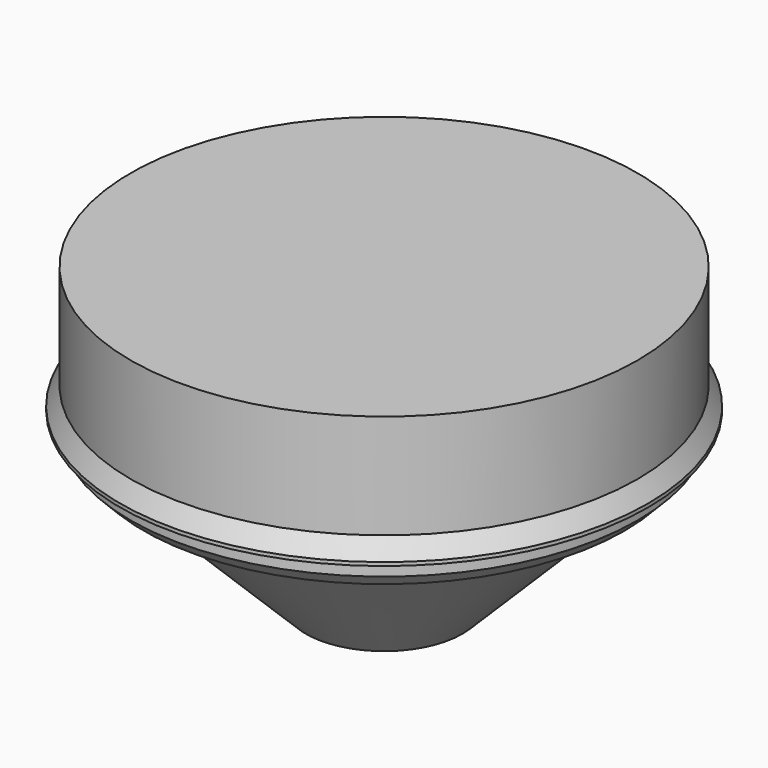
from build123d import *

# Parameters (mm, degrees)
F5_R      = 1.5
F6_DEPTH  = 5
F9_SCALE  = 1.5
F11_W     = 16
F11_H     = 14
F11_W_2   = 13
F11_H_2   = 7
F12_DEPTH = 25


with BuildPart() as f1:
    # F0 (on Front) → F1 (revolve)
    with BuildSketch(Plane.XZ):
        Polygon((30, 20), (10, 0), (14.2426406871, 0), (34.2426406871, 20), align=None)
        Polygon((14.2426406871, 0), (10, 0), (0, 0), (0, -3), (11.2426406871, -3), align=None)
    revolve(axis=Axis((0, 0, 22.637244314), (0, 0, 1)))


with BuildPart() as f4:
    # F2 (on Front) → F4 (revolve)
    with BuildSketch(Plane.XZ):
        Polygon((27.690468356, 20), (29.4864065244, 20), (29.6117793769, 20.1395396143), (34.3815907836, 20.1439280063), (34.3159139156, 19.9222583324), (33.2322780835, 18.8106978722), (34.4981237986, 17.5766527402), (36.3766141236, 19.503550604), (36.3766141236, 23.2204608619), (27.690468356, 23.2204608619), align=None)
        Polygon((27.690468356, 18.0011261255), (29.4864065244, 20), (27.690468356, 20), align=None)
    revolve(axis=Axis((0, 0, 19.0411023796), (0, 0, 1)))

    # F5 (on face) → F6 (cut)
    with BuildSketch(Plane.XY.offset(23.2204608619)):
        with Locations((0, 31.3766141236)):
            Circle(F5_R)
        with Locations((6.5235648946, 30.6909598241)):
            Circle(F5_R)
        with Locations((12.7620186997, 28.6639633088)):
            Circle(F5_R)
        with Locations((18.4427110487, 25.3842140519)):
            Circle(F5_R)
        with Locations((23.3173684269, 20.995052834)):
            Circle(F5_R)
        with Locations((27.1729449158, 15.6883070618)):
            Circle(F5_R)
        with Locations((31.2047297484, 3.2797492569)):
            Circle(F5_R)
        with Locations((31.2047297484, -3.2797492569)):
            Circle(F5_R)
        with Locations((29.8409333215, -9.6959069901)):
            Circle(F5_R)
        with Locations((-6.5235648946, 30.6909598241)):
            Circle(F5_R)
        with Locations((-12.7620186997, 28.6639633088)):
            Circle(F5_R)
        with Locations((-18.4427110487, 25.3842140519)):
            Circle(F5_R)
        with Locations((-23.3173684269, 20.995052834)):
            Circle(F5_R)
        with Locations((-29.8409333215, 9.6959069901)):
            Circle(F5_R)
        with Locations((-31.2047297484, 3.2797492569)):
            Circle(F5_R)
        with Locations((-31.2047297484, -3.2797492569)):
            Circle(F5_R)
        with Locations((-29.8409333215, -9.6959069901)):
            Circle(F5_R)
        with Locations((-27.1729449158, -15.6883070618)):
            Circle(F5_R)
        with Locations((-23.3173684269, -20.995052834)):
            Circle(F5_R)
        with Locations((-18.4427110487, -25.3842140519)):
            Circle(F5_R)
        with Locations((-12.7620186997, -28.6639633088)):
            Circle(F5_R)
        with Locations((-27.1729449158, 15.6883070618)):
            Circle(F5_R)
        with Locations((-6.5235648946, -30.6909598241)):
            Circle(F5_R)
        with Locations((0, -31.3766141236)):
            Circle(F5_R)
        with Locations((6.5235648946, -30.6909598241)):
            Circle(F5_R)
        with Locations((12.7620186997, -28.6639633088)):
            Circle(F5_R)
        with Locations((18.4427110487, -25.3842140519)):
            Circle(F5_R)
        with Locations((23.3173684269, -20.995052834)):
            Circle(F5_R)
        with Locations((27.1729449158, -15.6883070618)):
            Circle(F5_R)
        with Locations((29.8409333215, 9.6959069901)):
            Circle(F5_R)
    extrude(amount=-F6_DEPTH, mode=Mode.SUBTRACT)


with BuildPart() as f8:
    # F7 (on Front) → F8 (revolve)
    with BuildSketch(Plane.XZ):
        Polygon((34.8766141236, 23.2204608619), (36.3766141236, 23.2204608619), (36.3766141236, 24.7204608619), (36.3766141236, 39.7204608619), (0, 39.7204608619), (0, 38.2204608619), (34.8766141236, 38.2204608619), align=None)
        Polygon((36.3766141236, 24.7204608619), (36.3766141236, 23.2204608619), (36.3766141236, 21.6223846506), (37.8766141236, 21.6223846506), (37.8766141236, 22.1223846506), align=None)
    revolve(axis=Axis((0, 0, 19.0411023796), (0, 0, 1)))


with BuildPart() as f8_1:
    # F9: moved
    add(f8.part.scale(F9_SCALE))

    # F11 (on offset) → F12 (cut)
    with BuildSketch(Plane.YZ.offset(-60)):
        with Locations((-11.7728743628, 48.9317395091)):
            Rectangle(F11_W, F11_H)
        with Locations((10.1618623771, 52.0602014065)):
            Rectangle(F11_W_2, F11_H_2)
    extrude(amount=F12_DEPTH, mode=Mode.SUBTRACT)


with BuildPart() as f4_1:
    # F9: moved
    add(f4.part.scale(F9_SCALE))


with BuildPart() as f1_1:
    # F9: moved
    add(f1.part.scale(F9_SCALE))


solid = Compound([f8_1.part, f4_1.part, f1_1.part])
